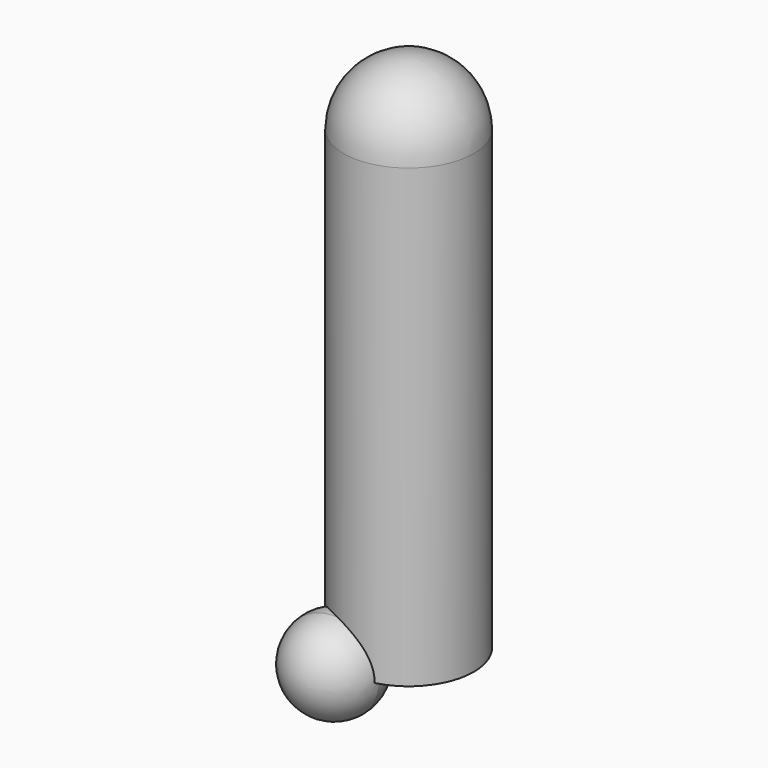
from build123d import *

# Parameters (mm, degrees)
F0_R     = 25.4
F1_DEPTH = 203.2
F2_R     = 25.4


with BuildPart() as f1:
    # F0 (on Top) → F1 (new body)
    with BuildSketch(Plane.XY):
        Circle(F0_R)
    extrude(amount=F1_DEPTH)

    # F2
    f2_edges = [f1.edges().sort_by_distance(p)[0] for p in [
        (-25.4, 0, 203.2),
    ]]
    fillet(f2_edges, radius=F2_R)

    # F3 (on Top) → F4 (revolve)
    with BuildSketch(Plane.XY):
        with BuildLine():
            ThreePointArc((-9.3745997379, -40.0344807354), (1.9888303668, -34.3120856795), (6.5670539636, -22.4413983524))
            ThreePointArc((6.5670539636, -22.4413983524), (0.7591214616, -9.34100212), (-12.8485319933, -4.8483159694))
            Line((-12.8485319933, -4.8483159694), (-11.1115658656, -22.4413983524))
            Line((-11.1115658656, -22.4413983524), (-9.3745997379, -40.0344807354))
        make_face()
    revolve(axis=Axis((-11.1115658656, -22.4413983524, 0), (0.0982523605, -0.9951615314, 0)))


solid = f1.part
